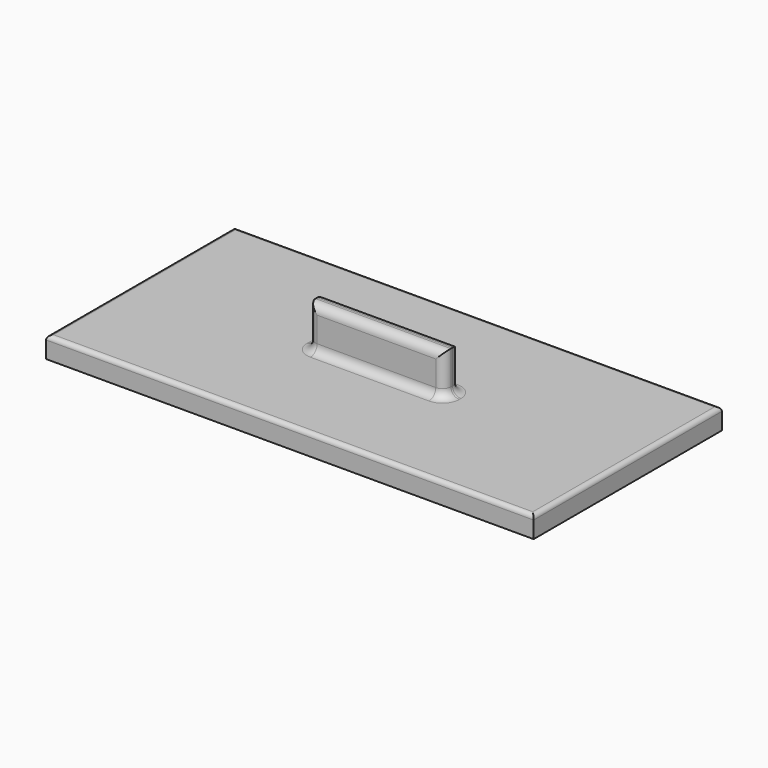
from build123d import *

# Parameters (mm, degrees)
F0_W     = 116
F0_H     = 56
F1_DEPTH = 5
F2_R     = 1
F3_W     = 32.2175696492
F3_H     = 4.4865976088
F4_DEPTH = 10
F5_F1_R  = 2
F5_F2_R  = 2


with BuildPart() as f1:
    # F0 (on Top) → F1 (new body)
    with BuildSketch(Plane.XY):
        Rectangle(F0_W, F0_H)
    extrude(amount=F1_DEPTH)

    # F2
    f2_edges = [f1.edges().sort_by_distance(p)[0] for p in [
        (0, -28, 5),
        (-58, 0, 5),
        (0, 28, 5),
        (58, 0, 5),
    ]]
    fillet(f2_edges, radius=F2_R)

    # F3 (on face) → F4 (join)
    with BuildSketch(Plane.XY.offset(5)):
        Rectangle(F3_W, F3_H)
    extrude(amount=F4_DEPTH)

    # F5: fillet of radius 2 on 8 edges, made by hand

    # F5_f1
    f5_f1_edges = [f1.edges().sort_by_distance(p)[0] for p in [
        (-16.1087848246, -2.2432988044, 10),
        (-16.1087848246, 2.2432988044, 10),
        (0, -2.2432988044, 15),
        (0, 2.2432988044, 15),
        (16.1087848246, -2.2432988044, 10),
        (16.1087848246, 2.2432988044, 10),
    ]]
    fillet(f5_f1_edges, radius=F5_F1_R)

    # F5_f2
    f5_f2_edges = [f1.edges().sort_by_distance(p)[0] for p in [
        (0, -2.2432988044, 5),
        (0, 2.2432988044, 5),
        (15.522998387, 1.6575123668, 5),
        (-15.522998387, 1.6575123668, 5),
        (-15.522998387, -1.6575123668, 5),
        (15.522998387, -1.6575123668, 5),
    ]]
    fillet(f5_f2_edges, radius=F5_F2_R)


solid = f1.part
